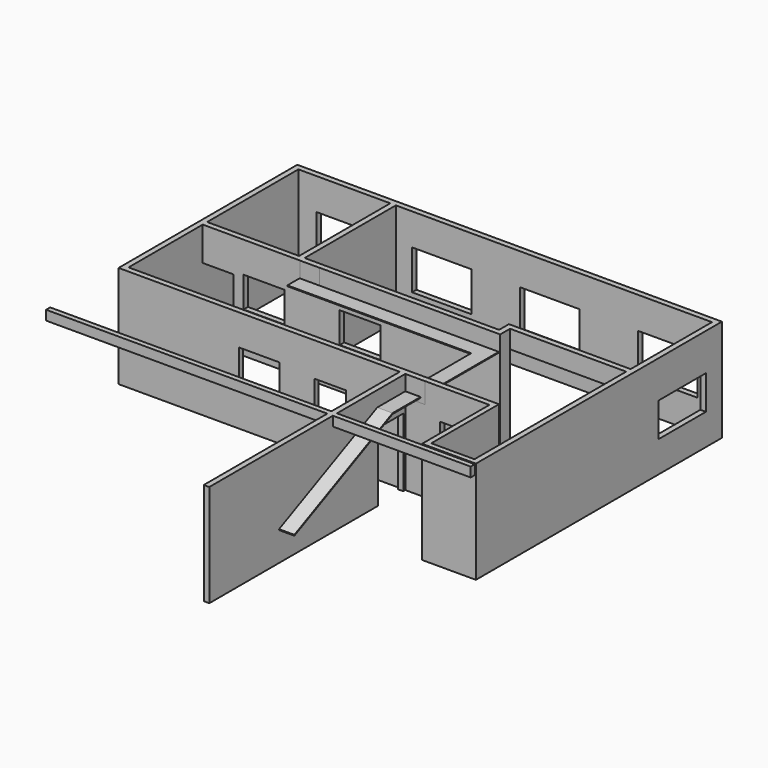
from build123d import *

# Parameters (mm, degrees)
F1_DEPTH  = 3054.35
F2_W      = 1219.2
F2_H      = 914.4
F3_DEPTH  = 165.1
F4_W      = 1778
F4_H      = 1181.1
F5_DEPTH  = 165.101
F6_W      = 1778
F6_H      = 1016
F7_DEPTH  = 165.101
F11_DEPTH = 3054.35
F12_W     = 3467.1
F12_H     = 2514.6
F13_DEPTH = 165.1
F14_W     = 952.5
F14_H     = 2044.7
F15_DEPTH = 165.1
F16_W     = 914.4
F16_H     = 1009.65
F17_DEPTH = 165.1
F18_W     = 952.5
F18_H     = 1009.65
F19_DEPTH = 165.1
F20_W     = 12674.6
F20_H     = 152.4
F21_DEPTH = 285.75
F22_W     = 1219.2
F22_H     = 1219.2
F22_H_2   = 914.4
F23_DEPTH = 165.1
F24_W     = 368.3
F24_H     = 2514.6
F25_DEPTH = 165.1
F26_W     = 165.1
F26_H     = 203.2
F27_DEPTH = 2514.6
F30_DEPTH = 25.4
F32_DEPTH = 457.2
F33_W     = 588.8758589745
F33_H     = 614.0316539764
F34_DEPTH = 2.54
F35_W     = 581.7451477051
F35_H     = 590.6585269928
F36_DEPTH = 2.54


with BuildPart() as f1:
    # F0 (on Top) → F1 (new body)
    with BuildSketch(Plane.XY):
        Polygon((-8071.8270324707, -464.391151869), (-8071.8270324707, 2939.208848131), (-5328.6270324707, 2939.208848131), (-5328.6270324707, -464.391151869), (-7157.4270324707, -464.391151869), (-7157.4270324707, -629.491151869), (-5163.5270324707, -629.491151869), (-4249.1270324707, -629.491151869), (805.4729675293, -629.491151869), (805.4729675293, -464.391151869), (640.3729675293, -464.391151869), (-4249.1270324707, -464.391151869), (-5163.5270324707, -464.391151869), (-5163.5270324707, 2939.208848131), (4272.5729675293, 2939.208848131), (4272.5729675293, 48.6404670191), (4272.5729675293, -116.4595329809), (4272.5729675293, -3398.091151869), (4272.5729675293, -5922.4400688171), (2983.5229675293, -5922.4400688171), (2983.5229675293, -3398.091151869), (-1442.4270324707, -3398.091151869), (-1442.4270324707, -3563.191151869), (157.7729675293, -3563.191151869), (157.7729675293, -10878.391151869), (322.8729675293, -10878.391151869), (322.8729675293, -3563.191151869), (2831.1229675293, -3563.191151869), (2831.1229675293, -6074.8400688171), (4437.6729675293, -6074.8400688171), (4437.6729675293, -3398.091151869), (4437.6729675293, 3104.308848131), (-8236.9270324707, 3104.308848131), (-8236.9270324707, -3563.191151869), (-2394.9270324707, -3563.191151869), (-2394.9270324707, -3398.091151869), (-8071.8270324707, -3398.091151869), (-8071.8270324707, -629.491151869), align=None)
    extrude(amount=F1_DEPTH)

    # F2 (on face) → F3 (cut, through all)
    with BuildSketch(Plane.XZ.offset(629.491151869)):
        with Locations((-6243.0270324707, 1676.4)):
            Rectangle(F2_W, F2_H)
        with Locations((-3372.8270324707, 1676.4)):
            Rectangle(F2_W, F2_H)
    extrude(amount=-F3_DEPTH, mode=Mode.SUBTRACT)

    # F4 (on face) → F5 (cut, through all)
    with BuildSketch(Plane.XZ.offset(-2939.208848131)):
        with Locations((-6636.7270324707, 1517.65)):
            Rectangle(F4_W, F4_H)
        with Locations((-3791.9270324707, 1517.65)):
            Rectangle(F4_W, F4_H)
        with Locations((-566.1270324707, 1517.65)):
            Rectangle(F4_W, F4_H)
        with Locations((2951.7729675293, 1517.65)):
            Rectangle(F4_W, F4_H)
    extrude(amount=-F5_DEPTH, mode=Mode.SUBTRACT)

    # F6 (on face) → F7 (cut, through all)
    with BuildSketch(Plane(origin=(4272.5729675293, 0, 0), x_dir=(0, -1, 0), z_dir=(-1, 0, 0))):
        with Locations((-1618.408848131, 1435.1)):
            Rectangle(F6_W, F6_H)
    extrude(amount=-F7_DEPTH, mode=Mode.SUBTRACT)

    # F10 (on Top) → F11 (join, through all)
    with BuildSketch(Plane.XY):
        Polygon((4272.5729675293, -96.091151869), (640.3729675293, -96.091151869), (640.3729675293, -464.391151869), (805.4729675293, -464.391151869), (805.4729675293, -261.191151869), (4272.5729675293, -261.191151869), align=None)
    extrude(amount=F11_DEPTH)

    # F12 (on face) → F13 (cut, through all)
    with BuildSketch(Plane.XZ.offset(261.191151869)):
        with Locations((2539.0229675293, 1257.3)):
            Rectangle(F12_W, F12_H)
    extrude(amount=-F13_DEPTH, mode=Mode.SUBTRACT)

    # F14 (on face) → F15 (cut, through all)
    with BuildSketch(Plane(origin=(157.7729675293, 0, 0), x_dir=(0, -1, 0), z_dir=(-1, 0, 0))):
        with Locations((4115.641151869, 1022.35)):
            Rectangle(F14_W, F14_H)
    extrude(amount=-F15_DEPTH, mode=Mode.SUBTRACT)

    # F16 (on face) → F17 (join)
    with BuildSketch(Plane.XZ.offset(629.491151869)):
        with Locations((-7614.6270324707, 2549.525)):
            Rectangle(F16_W, F16_H)
    extrude(amount=-F17_DEPTH)

    # F18 (on face) → F19 (join)
    with BuildSketch(Plane.XZ.offset(3563.191151869)):
        with Locations((-1918.6770324707, 2549.525)):
            Rectangle(F18_W, F18_H)
    extrude(amount=-F19_DEPTH)

    # F20 (on face) → F21 (join)
    with BuildSketch(Plane.XY.offset(3054.35)):
        with Locations((-1899.6270324707, -6192.091151869)):
            Rectangle(F20_W, F20_H)
    extrude(amount=-F21_DEPTH)

    # F22 (on face) → F23 (cut, through all)
    with BuildSketch(Plane.XZ.offset(3563.191151869)):
        with Locations((1967.5229675293, 1524)):
            Rectangle(F22_W, F22_H)
        with Locations((-4039.5770324707, 1676.4)):
            Rectangle(F22_W, F22_H_2)
    extrude(amount=-F23_DEPTH, mode=Mode.SUBTRACT)

    # F24 (on face) → F25 (cut, through all)
    with BuildSketch(Plane.YZ.offset(805.4729675293)):
        with Locations((-280.241151869, 1257.3)):
            Rectangle(F24_W, F24_H)
    extrude(amount=-F25_DEPTH, mode=Mode.SUBTRACT)

    # F26 (on face) → F27 (join, through all)
    with BuildSketch(Plane(origin=(0, 0, 2514.6), x_dir=(1, 0, 0), z_dir=(0, 0, -1))):
        with Locations((722.9229675293, 362.791151869)):
            Rectangle(F26_W, F26_H)
    extrude(amount=F27_DEPTH)


with BuildPart() as f30:
    # F29 (on offset) → F30 (new body)
    with BuildSketch(Plane.XY.offset(2597.15)):
        Polygon((322.8729675293, -649.5954301834), (-5163.5270324707, -649.5954301834), (-5163.5270324707, -1106.7954301834), (322.8729675293, -1106.7954301834), (322.8729675293, -4611.9954301834), (780.0729675293, -4611.9954301834), (780.0729675293, -649.5954301834), align=None)
    extrude(amount=-F30_DEPTH)


with BuildPart() as f32:
    # F31 (on face) → F32 (new body)
    with BuildSketch(Plane.YZ.offset(322.8729675293)):
        Polygon((-8275.1349264518, 863.6), (-4611.9954301834, 2571.75), (-4611.9954301834, 2597.15), (-8275.1349264518, 889), align=None)
    extrude(amount=F32_DEPTH)


with BuildPart() as f34:
    # F33 (on face) → F34 (new body)
    with BuildSketch(Plane.XZ.offset(3563.191151869)):
        with Locations((617.3108970165, 2747.3341730118)):
            Rectangle(F33_W, F33_H)
    extrude(amount=F34_DEPTH)


with BuildPart() as f36:
    # F35 (on face) → F36 (new body)
    with BuildSketch(Plane.XZ.offset(629.491151869)):
        with Locations((-4872.6544586182, 2759.0207365036)):
            Rectangle(F35_W, F35_H)
    extrude(amount=F36_DEPTH)


solid = Compound([f1.part, f30.part, f32.part, f34.part, f36.part])
